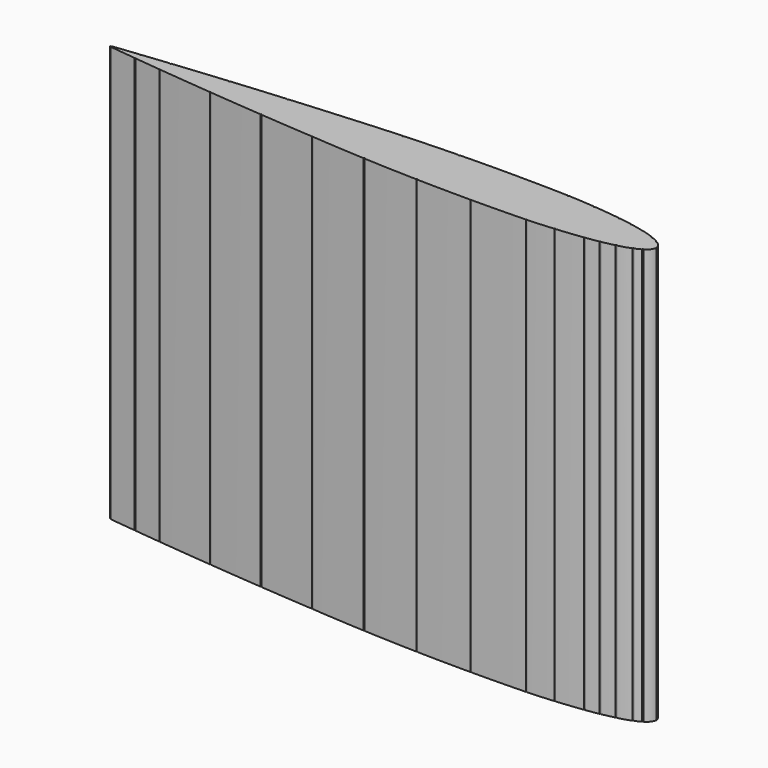
from build123d import *

# Parameters (mm, degrees)
F1_DEPTH = 762


# Not quite as in the source:
# - ends of sketch curves that miss each other by under 0.0002 mm in the source are joined


with BuildPart() as f1:
    # F0 (on Top) → F1 (new body)
    with BuildSketch(Plane.XY):
        with BuildLine():
            ThreePointArc((488.8742323068, 15.2944921486), (487.5203307918, 14.9025505993), (487.1193724988, 16.2538092487))
            ThreePointArc((487.1193724988, 16.2538092487), (481.824523523, 18.9352573397), (476.4205037428, 21.389266255))
            ThreePointArc((476.4205037428, 21.389266255), (475.1125647356, 20.8581030883), (474.5767217389, 22.1641318166))
            ThreePointArc((474.5767217389, 22.1641318166), (463.1842997703, 26.2876905948), (451.4772940324, 29.4081123545))
            ThreePointArc((451.4772940324, 29.4081123545), (450.276485478, 28.6452994006), (449.5280311535, 29.8551096795))
            ThreePointArc((449.5280311535, 29.8551096795), (438.0355044136, 32.4749833354), (426.4826400862, 34.8144778691))
            ThreePointArc((426.4826400862, 34.8144778691), (425.3154916622, 34.0171690515), (424.5169792351, 35.1834943482))
            ThreePointArc((424.5169792351, 35.1834943482), (413.0262686458, 37.1733622263), (401.4909912337, 38.8860732489))
            ThreePointArc((401.4909912337, 38.8860732489), (400.3671427029, 38.0288648232), (399.5087220344, 39.1517876884))
            ThreePointArc((399.5087220344, 39.1517876884), (375.5310617416, 42.0658475749), (351.4961188511, 44.4619816239))
            ThreePointArc((351.4961188511, 44.4619816239), (350.4124269023, 43.5538419038), (349.5038028578, 44.6371278018))
            ThreePointArc((349.5038028578, 44.6371278018), (325.5182950967, 46.4647415416), (301.4990594281, 47.7766380455))
            ThreePointArc((301.4990594281, 47.7766380455), (300.4634214455, 46.8206692193), (299.5004439239, 47.8497934687))
            ThreePointArc((299.5004439239, 47.8497934687), (250.4170586651, 48.9784061279), (201.3229831968, 49.4519342839))
            ThreePointArc((201.3229831968, 49.4519342839), (200.4972514489, 49.0200037773), (199.6739065342, 49.4564668725))
            ThreePointArc((199.6739065342, 49.4564668725), (150.5832624149, 49.2528772685), (101.4997048201, 48.3942955287))
            ThreePointArc((101.4997048201, 48.3942955287), (101.4999262023, 48.3821486609), (101.5, 48.37))
            ThreePointArc((101.5, 48.37), (100.5122846343, 47.370075459), (99.5003018245, 48.3454325854))
            ThreePointArc((99.5003018245, 48.3454325854), (50.4236366017, 46.8049664772), (1.3719002627, 44.6096835018))
            ThreePointArc((1.3719002627, 44.6096835018), (1.4674451568, 44.3730807552), (1.5, 44.12))
            ThreePointArc((1.5, 44.12), (0.297194356, 43.1407809894), (-0.4177397415, 44.5171822841))
            ThreePointArc((-0.4177397415, 44.5171822841), (-49.4818219256, 41.6405010198), (-98.503098248, 38.1086568293))
            ThreePointArc((-98.503098248, 38.1086568293), (-98.5007748622, 38.0693589124), (-98.5, 38.03))
            ThreePointArc((-98.5, 38.03), (-99.4653855857, 37.0305992584), (-100.4976036846, 37.9608126573))
            ThreePointArc((-100.4976036846, 37.9608126573), (-149.5105569813, 34.4207797542), (-198.5029069122, 30.606193006))
            ThreePointArc((-198.5029069122, 30.606193006), (-198.5007269923, 30.568124219), (-198.5, 30.53))
            ThreePointArc((-198.5, 30.53), (-199.4575267193, 29.5309023969), (-200.4963920408, 30.445130094))
            ThreePointArc((-200.4963920408, 30.445130094), (-249.5122047164, 26.3409146536), (-298.5042296621, 21.9618772772))
            ThreePointArc((-298.5042296621, 21.9618772772), (-298.5010579752, 21.915987292), (-298.5, 21.87))
            ThreePointArc((-298.5, 21.87), (-299.4539559536, 20.8710605895), (-300.4957598916, 21.7780095749))
            ThreePointArc((-300.4957598916, 21.7780095749), (-349.5135367847, 17.1080068146), (-398.5043233752, 12.1628873449))
            ThreePointArc((-398.5043233752, 12.1628873449), (-398.5010814285, 12.1164939523), (-398.5, 12.07))
            ThreePointArc((-398.5, 12.07), (-399.443021479, 11.0716245956), (-400.4935068963, 11.9562280921))
            ThreePointArc((-400.4935068963, 11.9562280921), (-424.5032598568, 9.4256444152), (-448.5059560316, 6.8289797637))
            ThreePointArc((-448.5059560316, 6.8289797637), (-448.5014901181, 6.7745711994), (-448.5, 6.72))
            ThreePointArc((-448.5, 6.72), (-449.4453720697, 5.7214932202), (-450.4940315785, 6.6109072825))
            ThreePointArc((-450.4940315785, 6.6109072825), (-474.5067314104, 3.9406998666), (-498.5119845054, 1.2043547292))
            ThreePointArc((-498.5119845054, 1.2043547292), (-498.5030006282, 1.1274096421), (-498.5, 1.05))
            ThreePointArc((-498.5, 1.05), (-499.2142366184, 0.0916997914), (-500.3366785795, 0.5023057837))
            ThreePointArc((-500.3366785795, 0.5023057837), (-500.458136, 0), (-500.3366785795, -0.5023057837))
            ThreePointArc((-500.3366785795, -0.5023057837), (-499.2142366184, -0.0916997914), (-498.5, -1.05))
            ThreePointArc((-498.5, -1.05), (-498.5030005898, -1.1274091465), (-498.5119843519, -1.2043537469))
            ThreePointArc((-498.5119843519, -1.2043537469), (-474.5067312795, -3.9406988813), (-450.49403147, -6.6109062944))
            ThreePointArc((-450.49403147, -6.6109062944), (-449.4453715735, -5.7214932474), (-448.5, -6.72))
            ThreePointArc((-448.5, -6.72), (-448.501490091, -6.7745707031), (-448.5059559233, -6.8289787756))
            ThreePointArc((-448.5059559233, -6.8289787756), (-424.5032597461, -9.425643427), (-400.4935067831, -11.9562271039))
            ThreePointArc((-400.4935067831, -11.9562271039), (-399.4430209825, -11.0716246239), (-398.5, -12.07))
            ThreePointArc((-398.5, -12.07), (-398.5010814054, -12.1164934555), (-398.5043232828, -12.1628863545))
            ThreePointArc((-398.5043232828, -12.1628863545), (-349.5135366927, -17.1080058236), (-300.4957598, -21.7780085834))
            ThreePointArc((-300.4957598, -21.7780085834), (-299.4539554563, -20.8710606125), (-298.5, -21.87))
            ThreePointArc((-298.5, -21.87), (-298.5010579523, -21.9159867947), (-298.5042295706, -21.9618762856))
            ThreePointArc((-298.5042295706, -21.9618762856), (-249.5122046283, -26.3409136613), (-200.4963919562, -30.4451291009))
            ThreePointArc((-200.4963919562, -30.4451291009), (-199.4575262213, -29.5309024181), (-198.5, -30.53))
            ThreePointArc((-198.5, -30.53), (-198.5007269733, -30.568123721), (-198.5029068362, -30.6061920122))
            ThreePointArc((-198.5029068362, -30.6061920122), (-149.5105569088, -34.4207787596), (-100.4976036156, -37.9608116621))
            ThreePointArc((-100.4976036156, -37.9608116621), (-99.4653850872, -37.0305992757), (-98.5, -38.03))
            ThreePointArc((-98.5, -38.03), (-98.5007748622, -38.0693589124), (-98.503098248, -38.1086568293))
            ThreePointArc((-98.503098248, -38.1086568293), (-49.4818219256, -41.6405010198), (-0.4177397415, -44.5171822841))
            ThreePointArc((-0.4177397415, -44.5171822841), (0.297194356, -43.1407809894), (1.5, -44.12))
            ThreePointArc((1.5, -44.12), (1.4674451568, -44.3730807552), (1.3719002627, -44.6096835018))
            ThreePointArc((1.3719002627, -44.6096835018), (50.4236366017, -46.8049664772), (99.5003018245, -48.3454325854))
            ThreePointArc((99.5003018245, -48.3454325854), (100.5122846343, -47.370075459), (101.5, -48.37))
            ThreePointArc((101.5, -48.37), (101.4999262023, -48.3821486609), (101.4997048201, -48.3942955287))
            ThreePointArc((101.4997048201, -48.3942955287), (150.5832624149, -49.2528772685), (199.6739065342, -49.4564668725))
            ThreePointArc((199.6739065342, -49.4564668725), (200.4972514489, -49.0200037773), (201.3229831968, -49.4519342839))
            ThreePointArc((201.3229831968, -49.4519342839), (250.4170586651, -48.9784061279), (299.5004439239, -47.8497934687))
            ThreePointArc((299.5004439239, -47.8497934687), (300.4634214455, -46.8206692193), (301.4990594281, -47.7766380455))
            ThreePointArc((301.4990594281, -47.7766380455), (325.5182950967, -46.4647415416), (349.5038028578, -44.6371278018))
            ThreePointArc((349.5038028578, -44.6371278018), (350.4124269023, -43.5538419038), (351.4961188511, -44.4619816239))
            ThreePointArc((351.4961188511, -44.4619816239), (375.5310617416, -42.0658475749), (399.5087220344, -39.1517876884))
            ThreePointArc((399.5087220344, -39.1517876884), (400.3671422118, -38.0288648891), (401.490991101, -38.886072267))
            ThreePointArc((401.490991101, -38.886072267), (413.0262684891, -37.1733612515), (424.5169790547, -35.1834933817))
            ThreePointArc((424.5169790547, -35.1834933817), (425.3154916626, -34.0171690514), (426.4826399039, -34.8144769037))
            ThreePointArc((426.4826399039, -34.8144769037), (438.035504208, -32.4749823797), (449.5280309249, -29.8551087345))
            ThreePointArc((449.5280309249, -29.8551087345), (450.2764859518, -28.645299292), (451.4772940324, -29.4081123545))
            ThreePointArc((451.4772940324, -29.4081123545), (463.1842997703, -26.2876905948), (474.5767217389, -22.1641318166))
            ThreePointArc((474.5767217389, -22.1641318166), (475.1125647356, -20.8581030883), (476.4205037428, -21.389266255))
            ThreePointArc((476.4205037428, -21.389266255), (481.824523523, -18.9352573397), (487.1193724988, -16.2538092487))
            ThreePointArc((487.1193724988, -16.2538092487), (487.5203307918, -14.9025505993), (488.8742323068, -15.2944921486))
            ThreePointArc((488.8742323068, -15.2944921486), (496.019452289, -9.0885932824), (500.3796021729, -0.6888050517))
            ThreePointArc((500.3796021729, -0.6888050517), (500.4696732905, -0.3496239971), (500.499999, 0))
            ThreePointArc((500.499999, 0), (500.4696732095, 0.3496244605), (500.379601649, 0.6888058734))
            ThreePointArc((500.379601649, 0.6888058734), (496.0194519925, 9.0885936587), (488.8742323068, 15.2944921486))
        make_face()
    extrude(amount=-F1_DEPTH)


solid = f1.part
